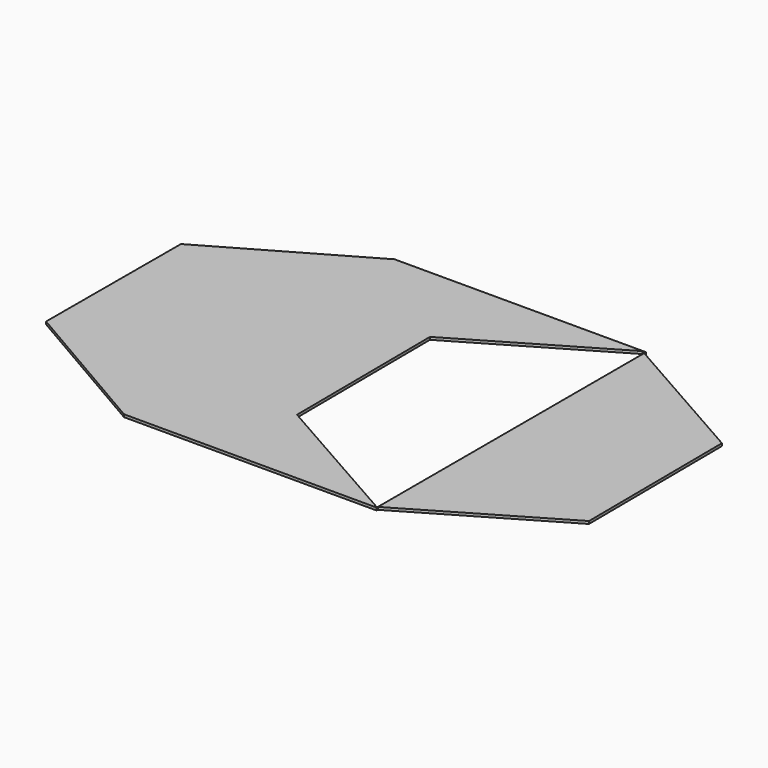
from build123d import *

# Parameters (mm, degrees)
F2_DEPTH = 1.27
F6_DEPTH = 1.27
F8_DEPTH = 1.27


with BuildPart() as f2:
    # F1 (on face) → F2 (new body)
    with BuildSketch(Plane.XY):
        Polygon((0, -0.3162004163), (-71.2728396538, -41.2281905004), (-71.4790315396, -123.6460217613), (-0.2061918858, -165.0335048029), (0, -164.9151466677), align=None)
    extrude(amount=F2_DEPTH)

    # F4 (on face) → F6 (join)
    with BuildSketch(Plane.XY):
        Polygon((51.3098860629, -41.7930965099), (122.2228978995, -0.1791509228), (122.7269796824, -0.4654425877), (122.7269796824, 0), (0, 0), (0, -165.1), (123.825, -165.1), (123.825, -164.361211811), (123.3873541232, -164.6180359287), (51.8921141747, -124.0125390129), align=None)
        Polygon((122.7269796824, 0), (122.7269796824, -0.4654425877), (123.825, -1.0890597775), (123.825, 0), align=None)
    extrude(amount=F6_DEPTH)


with BuildPart() as f8:
    # F7 (on face) → F8 (new body)
    with BuildSketch(Plane.XY):
        Polygon((123.825, -164.361211811), (194.3003659599, -123.0040903416), (193.718137848, -40.7846478386), (193.5964673758, -40.7155454761), (123.825, -1.0890597775), align=None)
    extrude(amount=F8_DEPTH)


solid = Compound([f2.part, f8.part])
